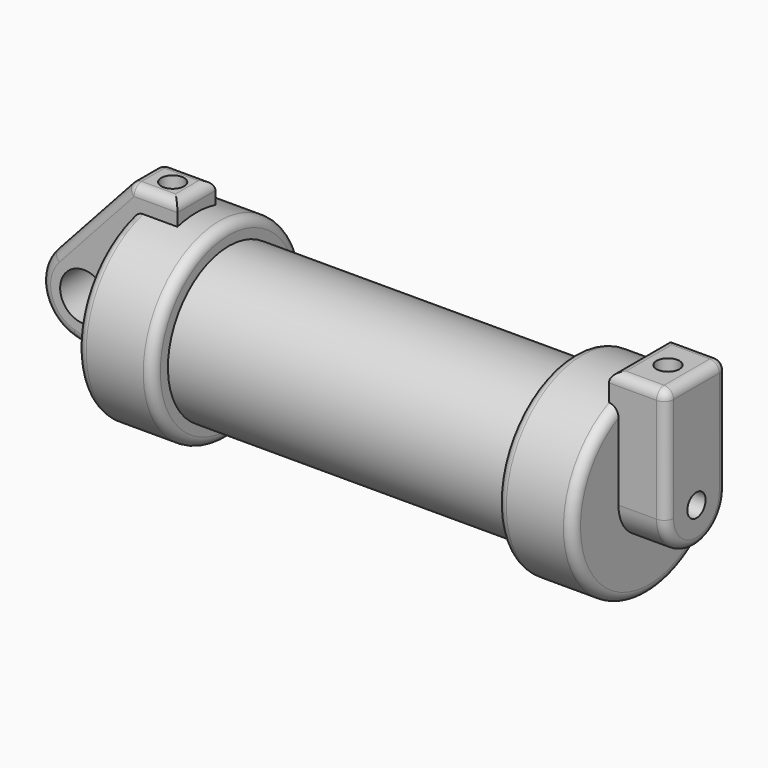
from build123d import *

# Parameters (mm, degrees)
F0_W          = 5.842
F0_H          = 12.7
F0_R          = 3.175
F2_DEPTH      = 3.175
F3_R          = 1.524
F4_DEPTH      = 1.27
F4_DEPTH_BACK = 6.35
F5_R          = 1.524
F6_DEPTH      = 10.414
F7_R          = 1.524
F8_DEPTH      = 17.78
F10_DEPTH     = 56.134
F11_R         = 1.27
F12_R         = 1.27
F13_T1_DEPTH  = 8.9637681337
F13_T3_DEPTH  = 12.7
F13_T5_DEPTH  = 3.81
F13_T10_DEPTH = 1.27
F13_T16_DEPTH = 1.27
F14_R         = 1.27
F15_R         = 1.27
F16_R         = 1.27


# Not quite as in the source:
# - a fillet or chamfer that OpenCascade refuses, or shapes differently, is made with other operations: its cross-section is extruded or revolved along the edge and cut away or added
# - the program builds the solid bodies; features that only make, move or delete a surface that nothing else refers to are left out


with BuildPart() as f1:
    # F0 (on Front) → F1 (revolve)
    with BuildSketch(Plane.XZ):
        Polygon((5.842, 12.7), (5.842, 0), (66.294, 0), (66.294, 12.7), (56.134, 12.7), (56.134, 10.16), (10.16, 10.16), (10.16, 12.7), align=None)
        with Locations((2.921, 6.35)):
            Rectangle(F0_W, F0_H)
    revolve(axis=Axis((33.147, 0, 0), (-1, 0, 0)))

    # F0 (on Front) → F2 (join, symmetric)
    with BuildSketch(Plane.XZ):
        with Locations((2.921, 6.35)):
            Rectangle(F0_W, F0_H)
        with BuildLine():
            Line((-0.9398, 0), (0, 0))
            Line((0, 0), (0, 12.7))
            Line((0, 12.7), (5.842, 12.7))
            Line((5.842, 12.7), (5.842, 15.24))
            Line((5.842, 15.24), (-0.508, 15.24))
            Line((-0.508, 15.24), (-10.8806298187, 3.8475430269))
            ThreePointArc((-10.8806298187, 3.8475430269), (-4.5919612295, 5.3297205562), (-0.9398, 0))
        make_face()
        with BuildLine():
            Line((5.842, 0), (0, 0))
            Line((0, 0), (-0.9398, 0))
            ThreePointArc((-0.9398, 0), (-3.1957909266, -4.5493385486), (-8.1826630726, -5.5069827884))
            Line((-8.1826630726, -5.5069827884), (5.842, -9.398))
            Line((5.842, -9.398), (5.842, 0))
        make_face()
        with BuildLine():
            ThreePointArc((-8.1826630726, -5.5069827884), (-3.1957909266, -4.5493385486), (-0.9398, 0))
            ThreePointArc((-0.9398, 0), (-4.5919612295, 5.3297205562), (-10.8806298187, 3.8475430269))
            ThreePointArc((-10.8806298187, 3.8475430269), (-12.1459778134, -1.5837270034), (-8.1826630726, -5.5069827884))
        make_face()
        with Locations((-6.6548, 0)):
            Circle(F0_R, mode=Mode.SUBTRACT)
    extrude(amount=F2_DEPTH, both=True)

    # F3 (on face) → F4 (join, two sides)
    with BuildSketch(Plane.YZ.offset(66.294)) as f4_sk:
        with BuildLine():
            ThreePointArc((-5.08, 0), (0, -5.08), (5.08, 0))
            ThreePointArc((5.08, 0), (0, 5.08), (-5.08, 0))
        make_face()
        Circle(F3_R, mode=Mode.SUBTRACT)
        with BuildLine():
            ThreePointArc((-5.08, 0), (0, 5.08), (5.08, 0))
            Line((5.08, 0), (5.08, 15.24))
            Line((5.08, 15.24), (-5.08, 15.24))
            Line((-5.08, 15.24), (-5.08, 0))
        make_face()
    extrude(amount=-F4_DEPTH)
    extrude(f4_sk.sketch, amount=F4_DEPTH_BACK)

    # F5 (on face) → F6 (cut)
    with BuildSketch(Plane.XY.offset(15.24)):
        with Locations((68.834, 0)):
            Circle(F5_R)
    extrude(amount=-F6_DEPTH, mode=Mode.SUBTRACT)

    # F7 (on face) → F8 (cut)
    with BuildSketch(Plane.XY.offset(15.24)):
        with Locations((2.667, 0)):
            Circle(F7_R)
    extrude(amount=-F8_DEPTH, mode=Mode.SUBTRACT)

    # F10 (cut, through all): a face of the model
    f10_faces = [f1.faces().sort_by_distance(p)[0] for p in [
        (66.294, 0, 0),
    ]]
    extrude(f10_faces, amount=-F10_DEPTH, mode=Mode.SUBTRACT)

    # F11
    f11_edges = [f1.edges().sort_by_distance(p)[0] for p in [
        (-12.145978, 3.175, -1.583727),
        (-5.694315, 3.175, 9.543772),
    ]]
    fillet(f11_edges, radius=F11_R)

    # F12
    f12_edges = [f1.edges().sort_by_distance(p)[0] for p in [
        (-5.694315, -3.175, 9.543772),
        (-12.145978, -3.175, -1.583727),
    ]]
    fillet(f12_edges, radius=F12_R)

    # F13: fillet of radius 1.27 on 3 edges, made by hand

    # F13_s2 → F13_t1 (cut)
    with BuildSketch(Plane.YZ.offset(0.0532318663)):
        with BuildLine():
            ThreePointArc((1.905, 15.24), (2.8030256121, 14.8680256121), (3.175, 13.97))
            Line((3.175, 13.97), (3.175, 15.24))
            Line((3.175, 15.24), (1.905, 15.24))
        make_face()
        with BuildLine():
            ThreePointArc((-1.905, 15.24), (-2.8030256121, 14.8680256121), (-3.175, 13.97))
            Line((-3.175, 13.97), (-3.175, 15.24))
            Line((-3.175, 15.24), (-1.905, 15.24))
        make_face()
    extrude(amount=F13_T1_DEPTH, mode=Mode.SUBTRACT)

    # F13_s4 → F13_t3 (cut)
    with BuildSketch(Plane.XZ.offset(-6.35)):
        with BuildLine():
            ThreePointArc((4.572, 15.24), (5.4700256121, 14.8680256121), (5.842, 13.97))
            Line((5.842, 13.97), (5.842, 15.24))
            Line((5.842, 15.24), (4.572, 15.24))
        make_face()
    extrude(amount=F13_T3_DEPTH, mode=Mode.SUBTRACT)

    # F13_s6 → F13_t5 (cut)
    with BuildSketch(Plane.XZ.offset(-1.905)):
        with BuildLine():
            ThreePointArc((0.0532318663, 15.24), (-0.4601090812, 15.1316286289), (-0.8858414267, 14.8250095615))
            Line((-0.8858414267, 14.8250095615), (-0.508, 15.24))
            Line((-0.508, 15.24), (0.0532318663, 15.24))
        make_face()
    extrude(amount=F13_T5_DEPTH, mode=Mode.SUBTRACT)


with BuildPart() as f13_tool8:
    # F13_s9 → F13_t10 (new body)
    with BuildSketch(Plane.XZ.offset(1.905)):
        Polygon((0.0532318663, 13.97), (0.0532318663, 15.24), (-0.508, 15.24), (-0.8858414267, 14.8250095615), align=None)
    extrude(amount=F13_T10_DEPTH)

    # F13_s11 → F13_t12 (revolve, cut)
    with BuildSketch(Plane(origin=(0.0532318663, -1.905, 13.97), x_dir=(0.4042054705, 0, -0.9146682118), z_dir=(-0.9146682118, 0, -0.4042054705))):
        with BuildLine():
            ThreePointArc((0, -1.27), (1.27, 0), (0, 1.27))
            Line((0, 1.27), (0, -1.27))
        make_face()
    revolve(axis=Axis((0.0532318663, -1.905, 13.97), (0, -1, 0)), mode=Mode.SUBTRACT)


with BuildPart() as f1_1:
    add(f1.part)

    # F13_t7: cut F13_tool8
    add(f13_tool8.part, mode=Mode.SUBTRACT)


with BuildPart() as f13_tool14:
    # F13_s15 → F13_t16 (new body)
    with BuildSketch(Plane.XZ.offset(-1.905)):
        Polygon((0.0532318663, 13.97), (0.0532318663, 15.24), (-0.508, 15.24), (-0.8858414267, 14.8250095615), align=None)
    extrude(amount=-F13_T16_DEPTH)

    # F13_s17 → F13_t18 (revolve, cut)
    with BuildSketch(Plane(origin=(0.0532318663, 1.905, 13.97), x_dir=(0.4042054705, 0, -0.9146682118), z_dir=(0.9146682118, 0, 0.4042054705))):
        with BuildLine():
            ThreePointArc((0, -1.27), (1.27, 0), (0, 1.27))
            Line((0, 1.27), (0, -1.27))
        make_face()
    revolve(axis=Axis((0.0532318663, 1.905, 13.97), (0, 1, 0)), mode=Mode.SUBTRACT)


with BuildPart() as f1_2:
    add(f1_1.part)

    # F13_t13: cut F13_tool14
    add(f13_tool14.part, mode=Mode.SUBTRACT)

    # F14
    f14_edges = [f1_2.edges().sort_by_distance(p)[0] for p in [
        (72.644, -5.08, 7.62),
        (68.834, -5.08, 15.24),
        (72.644, 0, -5.08),
        (72.644, 5.08, 7.62),
        (68.834, 5.08, 15.24),
        (72.644, 0, 15.24),
        (65.024, 0, 15.24),
    ]]
    fillet(f14_edges, radius=F14_R)

    # F15
    f15_edges = [f1_2.edges().sort_by_distance(p)[0] for p in [
        (66.294, 0, -12.7),
        (56.134, 0, -12.7),
    ]]
    fillet(f15_edges, radius=F15_R)

    # F16
    f16_edges = [f1_2.edges().sort_by_distance(p)[0] for p in [
        (10.16, 0, -12.7),
        (0, 0, -12.7),
    ]]
    fillet(f16_edges, radius=F16_R)


solid = f1_2.part
